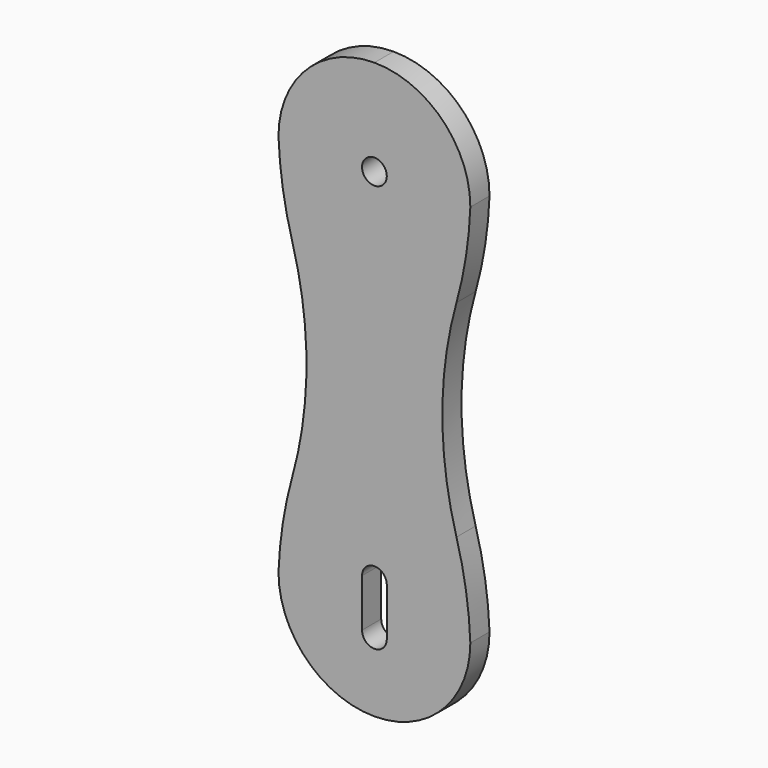
from build123d import *

# Parameters (mm, degrees)
F0_W        = 25.4
F0_H        = 76.2
F1_DEPTH    = 3.175
F2_R        = 1.6383
F3_DEPTH    = 25.4
F4_R        = 12.69999
F6_DEPTH    = 25.4
F7_T1_DEPTH = 34.92505


# Not quite as in the source:
# - a fillet or chamfer that OpenCascade refuses, or shapes differently, is made with other operations: its cross-section is extruded or revolved along the edge and cut away or added
# - a fillet or chamfer is up to 0.001 mm smaller than in the source, because OpenCascade refuses the exact size


with BuildPart() as f1:
    # F0 (on Front) → F1 (new body)
    with BuildSketch(Plane.XZ):
        with Locations((-15.0538895607, 2.5230566919)):
            Rectangle(F0_W, F0_H)
    extrude(amount=F1_DEPTH)

    # F2 (on face) → F3 (cut)
    with BuildSketch(Plane.XZ.offset(3.175)):
        with Locations((-15.0538895607, 27.9230566919)):
            Circle(F2_R)
        with BuildLine():
            ThreePointArc((-13.4155895607, -19.7019433081), (-15.0538895607, -18.0636433081), (-16.6921895607, -19.7019433081))
            Line((-16.6921895607, -19.7019433081), (-16.6921895607, -26.0519433081))
            ThreePointArc((-16.6921895607, -26.0519433081), (-15.0538895607, -27.6902433081), (-13.4155895607, -26.0519433081))
            Line((-13.4155895607, -26.0519433081), (-13.4155895607, -19.7019433081))
        make_face()
    extrude(amount=-F3_DEPTH, mode=Mode.SUBTRACT)

    # F4 (radius 12.7 in the source; OpenCascade refuses exactly that, so slightly less here)
    f4_edges = [f1.edges().sort_by_distance(p)[0] for p in [
        (-2.35389, -1.5875, -35.576943),
        (-27.75389, -1.5875, -35.576943),
        (-27.75389, -1.5875, 40.623057),
        (-2.35389, -1.5875, 40.623057),
    ]]
    fillet(f4_edges, radius=F4_R)

    # F5 (on face) → F6 (cut)
    with BuildSketch(Plane.XZ.offset(3.175)):
        with BuildLine():
            Line((-27.7538895607, 21.5730566919), (-27.7538895607, -16.5269433081))
            ThreePointArc((-27.7538895607, -16.5269433081), (-24.0467499538, 2.5230566919), (-27.7538895607, 21.5730566919))
        make_face()
        with BuildLine():
            Line((-2.3538895607, -16.5269433081), (-2.3538895607, 21.5730566919))
            ThreePointArc((-2.3538895607, 21.5730566919), (-6.0610291676, 2.5230566919), (-2.3538895607, -16.5269433081))
        make_face()
    extrude(amount=-F6_DEPTH, mode=Mode.SUBTRACT)

    # F7: fillet of radius 50.8 on 4 edges, made by hand

    # F7_s2 → F7_t1 (cut)
    with BuildSketch(Plane.XZ.offset(-15.875025)):
        with BuildLine():
            ThreePointArc((-27.7538895607, 27.9230666919), (-27.1805107314, 22.0006589845), (-25.9185762153, 16.1859192989))
            ThreePointArc((-25.9185762153, 16.1859192989), (-26.7607326385, 18.9052097481), (-27.7538895607, 21.5730566919))
            Line((-27.7538895607, 21.5730566919), (-27.7538895607, 27.9230666919))
        make_face()
        with BuildLine():
            ThreePointArc((-25.9185762153, -11.1398059151), (-27.1805107314, -16.9545456007), (-27.7538895607, -22.8769533081))
            Line((-27.7538895607, -22.8769533081), (-27.7538895607, -16.5269433081))
            ThreePointArc((-27.7538895607, -16.5269433081), (-26.7607326385, -13.8590963643), (-25.9185762153, -11.1398059151))
        make_face()
        with BuildLine():
            ThreePointArc((-2.3538895607, 27.9230666919), (-2.92726839, 22.0006589845), (-4.1892029061, 16.1859192989))
            ThreePointArc((-4.1892029061, 16.1859192989), (-3.3470464829, 18.9052097481), (-2.3538895607, 21.5730566919))
            Line((-2.3538895607, 21.5730566919), (-2.3538895607, 27.9230666919))
        make_face()
        with BuildLine():
            ThreePointArc((-4.1892029061, -11.1398059151), (-2.92726839, -16.9545456007), (-2.3538895607, -22.8769533081))
            Line((-2.3538895607, -22.8769533081), (-2.3538895607, -16.5269433081))
            ThreePointArc((-2.3538895607, -16.5269433081), (-3.3470464829, -13.8590963643), (-4.1892029061, -11.1398059151))
        make_face()
    extrude(amount=F7_T1_DEPTH, mode=Mode.SUBTRACT)


solid = f1.part
